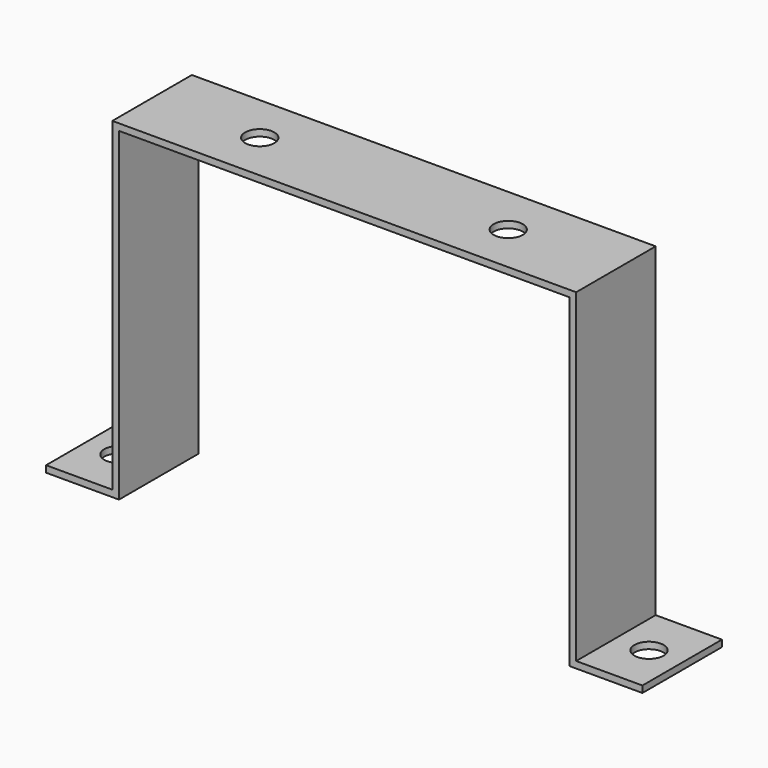
from build123d import *

# Parameters (mm, degrees)
F1_DEPTH = 30
F2_R     = 4.4
F3_R     = 4.4
F4_DEPTH = 25


# Not quite as in the source:
# - a feature names something its author has since deleted; it is built from what else it names


with BuildPart() as f1:
    # F0 (on Front) → F1 (new body)
    with BuildSketch(Plane.XZ):
        Polygon((90, -1), (90, 1), (70, 1), (70, 99), (-70, 99), (-70, 1), (-90, 1), (-90, -1), (-68, -1), (-68, 97), (68, 97), (68, -1), align=None)
    extrude(amount=F1_DEPTH)

    # F2 (on face) + F3 (on face) → F4 (cut)
    with BuildSketch(Plane.XY.offset(1)):
        with Locations((-80, -15)):
            Circle(F2_R)
        with Locations((80, -15)):
            Circle(F2_R)
    with BuildSketch(Plane.XY.offset(99)):
        with Locations((-37.5, -15)):
            Circle(F3_R)
        with Locations((37.5, -15)):
            Circle(F3_R)
    extrude(amount=-F4_DEPTH, mode=Mode.SUBTRACT)


solid = f1.part
